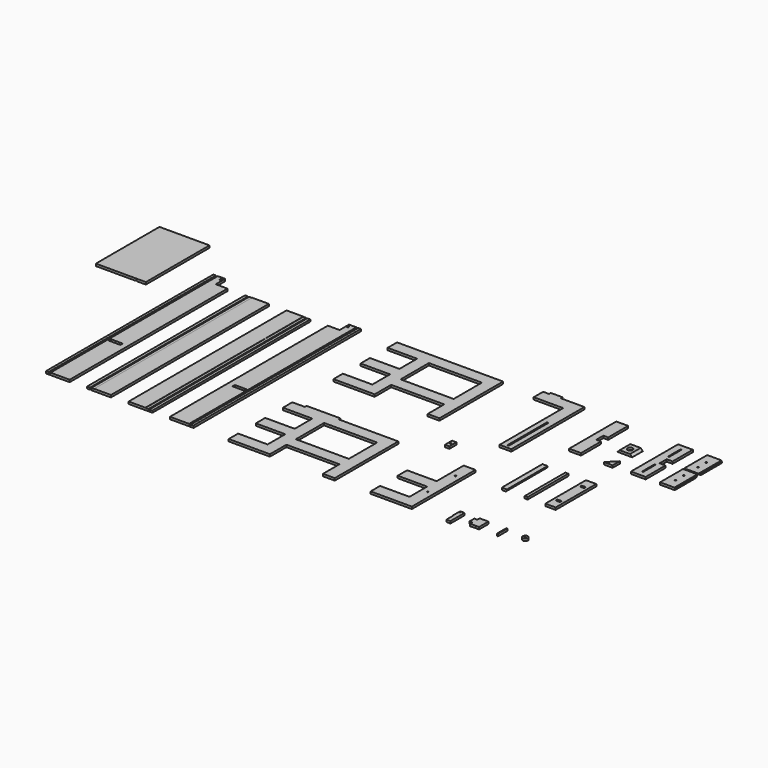
from build123d import *

# Parameters (mm, degrees)
F0_W      = 431.8
F0_H      = 685.8
F1_DEPTH  = 19.05
F0_W_2    = 457.2
F0_H_2    = 304.8
F0_R      = 6.35
F0_W_3    = 101.6
F0_H_3    = 25.4
F0_R_2    = 9.525
F0_W_4    = 205.0313949585
F0_H_4    = 1701.8
F0_W_5    = 38.1
F0_H_5    = 76.2
F0_R_3    = 4.7625
F0_W_6    = 127
F0_H_6    = 114.3
F0_R_4    = 22.225
F0_R_5    = 3.96875
F0_W_7    = 44.45
F0_H_7    = 438.15
F0_W_8    = 25.4
F0_W_9    = 88.9
F0_R_6    = 3.175
F0_W_10   = 7.9375
F0_H_8    = 101.6
F2_W      = 12.7
F2_H      = 685.8
F3_DEPTH  = 6.35
F4_W      = 15.875
F4_H      = 6.35
F5_DEPTH  = 2118.3410353432
F7_DEPTH  = 2118.3410353432
F9_DEPTH  = 2118.3410353432
F10_W     = 15.875
F10_H     = 6.35
F11_DEPTH = 2118.3410353432
F12_R     = 6.35
F13_DEPTH = 6.35
F15_DEPTH = 607.24668367
F16_W     = 3.175
F16_H     = 247.65
F16_R     = 6.35
F17_DEPTH = 6.35
F19_DEPTH = 127.001
F20_W     = 3.175
F20_H     = 247.65
F20_R     = 6.35
F21_DEPTH = 6.35
F23_DEPTH = 127.001
F25_DEPTH = 1528.3764581451
F27_DEPTH = 6.35
F28_R     = 5.55625
F29_DEPTH = 6.35
F30_R     = 3.96875
F31_DEPTH = 2048.008718277
F32_W     = 7.9375
F32_H     = 4.7625
F33_DEPTH = 2073.408718277


with BuildPart() as f1:
    # F0 (on Top) → F1 (new body)
    with BuildSketch(Plane.XY):
        with Locations((-215.9, -342.9)):
            Rectangle(F0_W, F0_H)
    extrude(amount=F1_DEPTH)

    # F2 (on face) → F3 (cut)
    with BuildSketch(Plane(origin=(0, 0, 0), x_dir=(1, 0, 0), z_dir=(0, 0, -1))):
        with Locations((-82.55, 342.9)):
            Rectangle(F2_W, F2_H)
    extrude(amount=-F3_DEPTH, mode=Mode.SUBTRACT)


with BuildPart() as f1b:
    # F0 (on Top) → F1, piece 2 (new body)
    with BuildSketch(Plane.XY):
        Polygon((2784.2749542236, -315.6766593456), (1869.8749542236, -315.6766593456), (1869.8749542236, -417.2766593456), (2123.8749542236, -417.2766593456), (2123.8749542236, -607.7766593456), (1869.8749542236, -607.7766593456), (1869.8749542236, -709.3766593456), (2123.8749542236, -709.3766593456), (2123.8749542236, -899.8766593456), (1869.8749542236, -899.8766593456), (1869.8749542236, -1001.4766593456), (2225.4749542236, -1001.4766593456), (2225.4749542236, -823.6766593456), (2682.6749542236, -823.6766593456), (2682.6749542236, -1001.4766593456), (2784.2749542236, -1001.4766593456), align=None)
        with Locations((2454.0749542236, -569.6766593456)):
            Rectangle(F0_W_2, F0_H_2, mode=Mode.SUBTRACT)
    extrude(amount=F1_DEPTH)


with BuildPart() as f1c:
    # F0 (on Top) → F1, piece 3 (new body)
    with BuildSketch(Plane.XY):
        Polygon((1972.5728313446, -1438.1806850433), (1864.6228313446, -1438.1806850433), (1864.6228313446, -1539.7806850433), (2118.6228313446, -1539.7806850433), (2118.6228313446, -1730.2806850433), (1864.6228313446, -1730.2806850433), (1864.6228313446, -1831.8806850433), (2118.6228313446, -1831.8806850433), (2118.6228313446, -2022.3806850433), (1864.6228313446, -2022.3806850433), (1864.6228313446, -2123.9806850433), (2220.2228313446, -2123.9806850433), (2220.2228313446, -1946.1806850433), (2677.4228313446, -1946.1806850433), (2677.4228313446, -2123.9806850433), (2779.0228313446, -2123.9806850433), (2779.0228313446, -1438.1806850433), (2264.6728313446, -1438.1806850433), (2264.6728313446, -1419.1306850433), (1972.5728313446, -1419.1306850433), align=None)
        with Locations((2448.8228313446, -1692.1806850433)):
            Rectangle(F0_W_2, F0_H_2, mode=Mode.SUBTRACT)
    extrude(amount=F1_DEPTH)


with BuildPart() as f1d:
    # F0 (on Top) → F1, piece 4 (new body)
    with BuildSketch(Plane.XY):
        Polygon((3138.8670032501, -263.583958149), (3088.0670032501, -263.583958149), (3088.0670032501, -365.183958149), (3342.0670032501, -365.183958149), (3342.0670032501, -1050.983958149), (3443.6670032501, -1050.983958149), (3443.6670032501, -263.583958149), (3240.4670032501, -263.583958149), (3240.4670032501, -244.533958149), (3138.8670032501, -244.533958149), align=None)
        with BuildLine():
            Line((3386.5170032501, -1019.233958149), (3386.5170032501, -600.133958149))
            ThreePointArc((3386.5170032501, -600.133958149), (3388.3768751896, -595.6438300884), (3392.8670032501, -593.783958149))
            ThreePointArc((3392.8670032501, -593.783958149), (3397.3571313107, -595.6438300884), (3399.2170032501, -600.133958149))
            Line((3399.2170032501, -600.133958149), (3399.2170032501, -1019.233958149))
            ThreePointArc((3399.2170032501, -1019.233958149), (3397.3571313107, -1023.7240862095), (3392.8670032501, -1025.583958149))
            ThreePointArc((3392.8670032501, -1025.583958149), (3388.3768751896, -1023.7240862095), (3386.5170032501, -1019.233958149))
        make_face(mode=Mode.SUBTRACT)
    extrude(amount=F1_DEPTH)


with BuildPart() as f1e:
    # F0 (on Top) → F1, piece 5 (new body)
    with BuildSketch(Plane.XY):
        Polygon((3443.6670032501, -2123.6350973129), (3443.6670032501, -1437.8350973129), (3342.0670032501, -1437.8350973129), (3342.0670032501, -1729.9350973129), (3088.0670032501, -1729.9350973129), (3088.0670032501, -1831.5350973129), (3342.0670032501, -1831.5350973129), (3342.0670032501, -2022.0350973129), (3088.0670032501, -2022.0350973129), (3088.0670032501, -2123.6350973129), align=None)
        with Locations((3392.8670032501, -1888.6850973129)):
            Circle(F0_R, mode=Mode.SUBTRACT)
        with Locations((3392.8670032501, -1590.2350973129)):
            Circle(F0_R, mode=Mode.SUBTRACT)
    extrude(amount=F1_DEPTH)


with BuildPart() as f1f:
    # F0 (on Top) → F1, piece 6 (new body)
    with BuildSketch(Plane.XY):
        Polygon((386.8345108986, -314.9400353432), (285.2345108986, -314.9400353432), (285.2345108986, -2118.3400353432), (488.4345108986, -2118.3400353432), (488.4345108986, -416.5400353432), (386.8345108986, -416.5400353432), align=None)
        with Locations((386.6274400234, -1496.0400353432)):
            Rectangle(F0_W_3, F0_H_3, mode=Mode.SUBTRACT)
        with Locations((374.1345108986, -343.5150353432)):
            Circle(F0_R_2, mode=Mode.SUBTRACT)
    extrude(amount=F1_DEPTH)

    # F4 (on face) → F5 (cut, through all)
    with BuildSketch(Plane.XZ.offset(2118.3400353432)):
        with Locations((315.3970108986, 15.875)):
            Rectangle(F4_W, F4_H)
    extrude(amount=-F5_DEPTH, mode=Mode.SUBTRACT)


with BuildPart() as f1g:
    # F0 (on Top) → F1, piece 7 (new body)
    with BuildSketch(Plane.XY):
        with Locations((742.2453165054, -1267.4400353432)):
            Rectangle(F0_W_4, F0_H_4)
    extrude(amount=F1_DEPTH)

    # F6 (on face) → F7 (cut, through all)
    with BuildSketch(Plane.XZ.offset(2118.3400353432)):
        Polygon((700.0546190262, 19.05), (639.7296190262, 19.05), (639.7296190262, 17.4625), (665.1296190262, 17.4625), (665.1296190262, 0), (674.6546190262, 0), (674.6546190262, 17.4625), (700.0546190262, 17.4625), align=None)
    extrude(amount=-F7_DEPTH, mode=Mode.SUBTRACT)


with BuildPart() as f1h:
    # F0 (on Top) → F1, piece 8 (new body)
    with BuildSketch(Plane.XY):
        Polygon((1455.0875170708, -314.9400353432), (1455.0875170708, -416.5400353432), (1353.4875170708, -416.5400353432), (1353.4875170708, -2118.3400353432), (1556.6875170708, -2118.3400353432), (1556.6875170708, -314.9400353432), align=None)
        with Locations((1455.2945879459, -1496.0400353432)):
            Rectangle(F0_W_3, F0_H_3, mode=Mode.SUBTRACT)
        with Locations((1467.7875170708, -343.5150353432)):
            Circle(F0_R_2, mode=Mode.SUBTRACT)
    extrude(amount=F1_DEPTH)

    # F10 (on face) → F11 (cut, through all)
    with BuildSketch(Plane.XZ.offset(2118.3400353432)):
        with Locations((1526.5250170708, 15.875)):
            Rectangle(F10_W, F10_H)
    extrude(amount=-F11_DEPTH, mode=Mode.SUBTRACT)


with BuildPart() as f1i:
    # F0 (on Top) → F1, piece 9 (new body)
    with BuildSketch(Plane.XY):
        with Locations((1099.6767114639, -1267.4400353432)):
            Rectangle(F0_W_4, F0_H_4)
    extrude(amount=F1_DEPTH)

    # F8 (on face) → F9 (cut, through all)
    with BuildSketch(Plane.XZ.offset(2118.3400353432)):
        Polygon((1202.1924089432, 17.4625), (1202.1924089432, 19.05), (1141.8674089432, 19.05), (1141.8674089432, 17.4625), (1167.2674089432, 17.4625), (1167.2674089432, 0), (1176.7924089432, 0), (1176.7924089432, 17.4625), align=None)
    extrude(amount=-F9_DEPTH, mode=Mode.SUBTRACT)


with BuildPart() as f1j:
    # F0 (on Top) → F1, piece 10 (new body)
    with BuildSketch(Plane.XY):
        with Locations((3073.241827774, -1241.6836065292)):
            Rectangle(F0_W_5, F0_H_5)
        with Locations((3073.241827774, -1241.6836065292)):
            Circle(F0_R_3, mode=Mode.SUBTRACT)
    extrude(amount=F1_DEPTH)

    # F12 (on face) → F13 (cut)
    with BuildSketch(Plane.XY.offset(19.05)):
        with Locations((3073.241827774, -1241.6836065292)):
            Circle(F12_R)
    extrude(amount=-F13_DEPTH, mode=Mode.SUBTRACT)


with BuildPart() as f1k:
    # F0 (on Top) → F1, piece 11 (new body)
    with BuildSketch(Plane.XY):
        Polygon((3845.7095623016, -294.3373322487), (3743.0131435394, -294.3373322487), (3743.0131435394, -802.3373322487), (3845.7095623016, -802.3373322487), (3845.7095623016, -586.4373322487), (3804.2194843292, -586.4373322487), (3804.2194843292, -510.2373322487), (3845.7095623016, -510.2373322487), align=None)
    extrude(amount=F1_DEPTH)


with BuildPart() as f1l:
    # F0 (on Top) → F1, piece 12 (new body)
    with BuildSketch(Plane.XY):
        with Locations((4067.4343833923, -550.09568367)):
            Rectangle(F0_W_6, F0_H_6)
        with Locations((4067.4343833923, -550.09568367)):
            Circle(F0_R_4, mode=Mode.SUBTRACT)
    extrude(amount=F1_DEPTH)

    # F14 (on face) → F15 (cut, through all)
    with BuildSketch(Plane.XZ.offset(607.24568367)):
        Polygon((4003.9343833923, 19.05), (4003.9343833923, 0), (4022.9843833923, 19.05), align=None)
        Polygon((4111.8843833923, 19.05), (4130.9343833923, 0), (4130.9343833923, 19.05), align=None)
    extrude(amount=-F15_DEPTH, mode=Mode.SUBTRACT)


with BuildPart() as f1m:
    # F0 (on Top) → F1, piece 13 (new body)
    with BuildSketch(Plane.XY):
        Polygon((4403.0815620422, -294.3373322487), (4276.0815620422, -294.3373322487), (4276.0815620422, -802.3373322487), (4403.0815620422, -802.3373322487), (4403.0815620422, -588.3157849312), (4352.2815620422, -588.3157849312), (4352.2815620422, -512.1157849312), (4403.0815620422, -512.1157849312), align=None)
        with BuildLine():
            Line((4344.3440620422, -624.5373322487), (4344.3440620422, -751.5373322487))
            ThreePointArc((4344.3440620422, -751.5373322487), (4339.5815620422, -756.2998322487), (4334.8190620422, -751.5373322487))
            Line((4334.8190620422, -751.5373322487), (4334.8190620422, -624.5373322487))
            ThreePointArc((4334.8190620422, -624.5373322487), (4339.5815620422, -619.7748322487), (4344.3440620422, -624.5373322487))
        make_face(mode=Mode.SUBTRACT)
        with BuildLine():
            Line((4344.3440620422, -345.1373322487), (4344.3440620422, -472.1373322487))
            ThreePointArc((4344.3440620422, -472.1373322487), (4339.5815620422, -476.8998322487), (4334.8190620422, -472.1373322487))
            Line((4334.8190620422, -472.1373322487), (4334.8190620422, -345.1373322487))
            ThreePointArc((4334.8190620422, -345.1373322487), (4339.5815620422, -340.3748322487), (4344.3440620422, -345.1373322487))
        make_face(mode=Mode.SUBTRACT)
    extrude(amount=F1_DEPTH)


with BuildPart() as f1n:
    # F0 (on Top) → F1, piece 14 (new body)
    with BuildSketch(Plane.XY):
        Polygon((4654.2750854492, -294.3373322487), (4527.2750854492, -294.3373322487), (4527.2750854492, -541.9873322487), (4651.1000854492, -541.9873322487), (4654.2750854492, -538.8123322487), align=None)
        with Locations((4590.7750854492, -472.1373322487)):
            Circle(F0_R_5, mode=Mode.SUBTRACT)
        with Locations((4590.7750854492, -383.2373322487)):
            Circle(F0_R_5, mode=Mode.SUBTRACT)
    extrude(amount=F1_DEPTH)

    # F16 (on face) → F17 (cut)
    with BuildSketch(Plane.XY.offset(19.05)):
        with Locations((4652.6875854492, -418.1623322487)):
            Rectangle(F16_W, F16_H)
        with Locations((4590.7750854492, -383.2373322487)):
            Circle(F16_R)
        with Locations((4590.7750854492, -472.1373322487)):
            Circle(F16_R)
    extrude(amount=-F17_DEPTH, mode=Mode.SUBTRACT)

    # F18 (on face) → F19 (cut, through all)
    with BuildSketch(Plane(origin=(4527.2750854492, 0, 0), x_dir=(0, -1, 0), z_dir=(-1, 0, 0))):
        Polygon((541.9873322487, 0), (541.9873322487, 19.05), (522.9373322487, 0), align=None)
    extrude(amount=-F19_DEPTH, mode=Mode.SUBTRACT)


with BuildPart() as f1o:
    # F0 (on Top) → F1, piece 15 (new body)
    with BuildSketch(Plane.XY):
        with Locations((3765.3821483612, -1309.3004581451)):
            Rectangle(F0_W_7, F0_H_7)
    extrude(amount=F1_DEPTH)

    # F24 (on face) → F25 (cut, through all)
    with BuildSketch(Plane.XZ.offset(1528.3754581451)):
        Polygon((3787.6071483612, 0), (3787.6071483612, 9.525), (3778.0821483612, 0), align=None)
    extrude(amount=-F25_DEPTH, mode=Mode.SUBTRACT)


with BuildPart() as f1p:
    # F0 (on Top) → F1, piece 16 (new body)
    with BuildSketch(Plane.XY):
        with Locations((3953.4577514648, -1309.3004581451)):
            Rectangle(F0_W_8, F0_H_7)
    extrude(amount=F1_DEPTH)


with BuildPart() as f1q:
    # F0 (on Top) → F1, piece 17 (new body)
    with BuildSketch(Plane.XY):
        with Locations((4162.9402191162, -1309.3004581451)):
            Rectangle(F0_W_9, F0_H_7)
        with BuildLine():
            ThreePointArc((4173.4103263855, -1434.7129581451), (4178.1728263855, -1439.4754581451), (4173.4103263855, -1444.2379581451))
            Line((4173.4103263855, -1444.2379581451), (4152.4701118469, -1444.2379581451))
            ThreePointArc((4152.4701118469, -1444.2379581451), (4147.7076118469, -1439.4754581451), (4152.4701118469, -1434.7129581451))
            Line((4152.4701118469, -1434.7129581451), (4173.4103263855, -1434.7129581451))
        make_face(mode=Mode.SUBTRACT)
        with BuildLine():
            Line((4173.4103263855, -1183.8879581451), (4152.4701118469, -1183.8879581451))
            ThreePointArc((4152.4701118469, -1183.8879581451), (4147.7076118469, -1179.1254581451), (4152.4701118469, -1174.3629581451))
            Line((4152.4701118469, -1174.3629581451), (4173.4103263855, -1174.3629581451))
            ThreePointArc((4173.4103263855, -1174.3629581451), (4178.1728263855, -1179.1254581451), (4173.4103263855, -1183.8879581451))
        make_face(mode=Mode.SUBTRACT)
    extrude(amount=F1_DEPTH)

    # F26 (on face) → F27 (cut)
    with BuildSketch(Plane.XY.offset(19.05)):
        with BuildLine():
            Line((4173.4103263855, -1169.6004581451), (4152.4701118469, -1169.6004581451))
            ThreePointArc((4152.4701118469, -1169.6004581451), (4142.9451118469, -1179.1254581451), (4152.4701118469, -1188.6504581451))
            Line((4152.4701118469, -1188.6504581451), (4173.4103263855, -1188.6504581451))
            ThreePointArc((4173.4103263855, -1188.6504581451), (4182.9353263855, -1179.1254581451), (4173.4103263855, -1169.6004581451))
        make_face()
        with BuildLine():
            Line((4173.4103263855, -1429.9504581451), (4152.4701118469, -1429.9504581451))
            ThreePointArc((4152.4701118469, -1429.9504581451), (4142.9451118469, -1439.4754581451), (4152.4701118469, -1449.0004581451))
            Line((4152.4701118469, -1449.0004581451), (4173.4103263855, -1449.0004581451))
            ThreePointArc((4173.4103263855, -1449.0004581451), (4182.9353263855, -1439.4754581451), (4173.4103263855, -1429.9504581451))
        make_face()
    extrude(amount=-F27_DEPTH, mode=Mode.SUBTRACT)


with BuildPart() as f1r:
    # F0 (on Top) → F1, piece 18 (new body)
    with BuildSketch(Plane.XY):
        with BuildLine():
            Line((3778.3746677399, -2125.7971256256), (3778.3746677399, -1973.3971256256))
            Line((3778.3746677399, -1973.3971256256), (3746.6246677399, -1973.3971256256))
            ThreePointArc((3746.6246677399, -1973.3971256256), (3742.1345396793, -1975.2569975651), (3740.2746677399, -1979.7471256256))
            Line((3740.2746677399, -1979.7471256256), (3740.2746677399, -2049.5971256256))
            Line((3740.2746677399, -2049.5971256256), (3743.4496677399, -2049.5971256256))
            Line((3743.4496677399, -2049.5971256256), (3743.4496677399, -2125.7971256256))
            Line((3743.4496677399, -2125.7971256256), (3778.3746677399, -2125.7971256256))
        make_face()
        with Locations((3748.2121677399, -1986.0971256256)):
            Circle(F0_R_6, mode=Mode.SUBTRACT)
    extrude(amount=F1_DEPTH)


with BuildPart() as f1s:
    # F0 (on Top) → F1, piece 19 (new body)
    with BuildSketch(Plane.XY):
        Polygon((3982.8455364227, -2073.407718277), (3982.8455364227, -1971.807718277), (3906.6455364227, -1971.807718277), (3906.6455364227, -1997.207718277), (3881.2455364227, -1997.207718277), (3881.2455364227, -2048.007718277), (3906.6455364227, -2048.007718277), (3906.6455364227, -2073.407718277), align=None)
        with Locations((3952.6830364227, -2022.607718277)):
            Circle(F0_R_6, mode=Mode.SUBTRACT)
    extrude(amount=F1_DEPTH)

    # F30 (on face) → F31 (cut, through all)
    with BuildSketch(Plane.XZ.offset(2048.007718277)):
        with Locations((3893.9455364227, 9.525)):
            Circle(F30_R)
    extrude(amount=-F31_DEPTH, mode=Mode.SUBTRACT)

    # F32 (on face) → F33 (cut, through all)
    with BuildSketch(Plane.XZ.offset(2073.407718277)):
        with Locations((3952.6830364227, 2.38125)):
            Rectangle(F32_W, F32_H)
    extrude(amount=-F33_DEPTH, mode=Mode.SUBTRACT)


with BuildPart() as f1t:
    # F0 (on Top) → F1, piece 20 (new body)
    with BuildSketch(Plane.XY):
        with Locations((4140.9521446228, -2022.1096618652)):
            Rectangle(F0_W_10, F0_H_8)
        with Locations((4140.9521446228, -2022.1096618652)):
            Circle(F0_R_6, mode=Mode.SUBTRACT)
    extrude(amount=F1_DEPTH)


with BuildPart() as f1u:
    # F0 (on Top) → F1, piece 21 (new body)
    with BuildSketch(Plane.XY):
        with Locations((4318.4003829956, -1993.5290813446)):
            Circle(F0_R_4)
        with Locations((4318.4003829956, -1993.5290813446)):
            Circle(F0_R_3, mode=Mode.SUBTRACT)
    extrude(amount=F1_DEPTH)

    # F28 (on face) → F29 (cut)
    with BuildSketch(Plane.XY.offset(19.05)):
        with Locations((4318.4003829956, -1993.5290813446)):
            Circle(F28_R)
    extrude(amount=-F29_DEPTH, mode=Mode.SUBTRACT)


with BuildPart() as f1v:
    # F0 (on Top) → F1, piece 22 (new body)
    with BuildSketch(Plane.XY):
        Polygon((4123.8512908936, -808.8287115097), (4123.8512908936, -732.6287115097), (4047.6512908936, -808.8287115097), align=None)
    extrude(amount=F1_DEPTH)


with BuildPart() as f1w:
    # F0 (on Top) → F1, piece 23 (new body)
    with BuildSketch(Plane.XY):
        Polygon((4654.2750854492, -802.3373322487), (4654.2750854492, -557.8623322487), (4651.1000854492, -554.6873322487), (4527.2750854492, -554.6873322487), (4527.2750854492, -802.3373322487), align=None)
        with Locations((4590.7750854492, -713.4373322487)):
            Circle(F0_R_5, mode=Mode.SUBTRACT)
        with Locations((4590.7750854492, -624.5373322487)):
            Circle(F0_R_5, mode=Mode.SUBTRACT)
    extrude(amount=F1_DEPTH)

    # F20 (on face) → F21 (cut)
    with BuildSketch(Plane.XY.offset(19.05)):
        with Locations((4652.6875854492, -678.5123322487)):
            Rectangle(F20_W, F20_H)
        with Locations((4590.7750854492, -624.5373322487)):
            Circle(F20_R)
        with Locations((4590.7750854492, -713.4373322487)):
            Circle(F20_R)
    extrude(amount=-F21_DEPTH, mode=Mode.SUBTRACT)

    # F22 (on face) → F23 (cut, through all)
    with BuildSketch(Plane(origin=(4527.2750854492, 0, 0), x_dir=(0, -1, 0), z_dir=(-1, 0, 0))):
        Polygon((554.6873322487, 19.05), (554.6873322487, 0), (573.7373322487, 0), align=None)
    extrude(amount=-F23_DEPTH, mode=Mode.SUBTRACT)


solid = Compound([f1.part, f1b.part, f1c.part, f1d.part, f1e.part, f1f.part, f1g.part, f1h.part, f1i.part, f1j.part, f1k.part, f1l.part, f1m.part, f1n.part, f1o.part, f1p.part, f1q.part, f1r.part, f1s.part, f1t.part, f1u.part, f1v.part, f1w.part])
